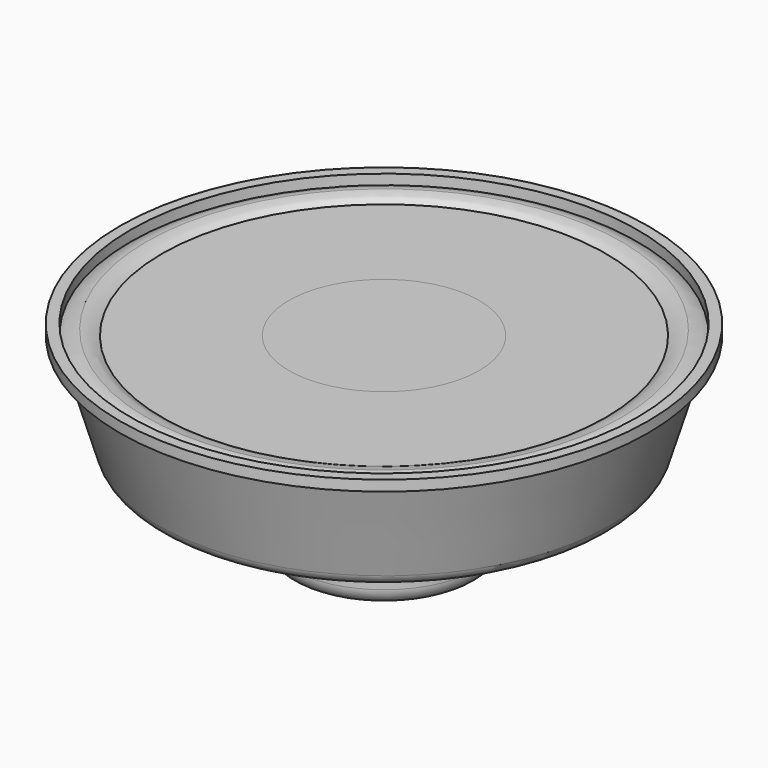
from build123d import *

# Parameters (mm, degrees)
F0_R     = 25
F0_R_2   = 24
F1_DEPTH = 1
F0_R_3   = 9
F2_DEPTH = 18
F0_R_4   = 21
F3_DEPTH = 10
F4_DEPTH = 0.5
F5_SIZE2 = 2.99999
F5_SIZE  = 9.99999
F6_R     = 1.5
F6_2_R   = 1.5


# Not quite as in the source:
# - a fillet or chamfer that OpenCascade refuses, or shapes differently, is made with other operations: its cross-section is extruded or revolved along the edge and cut away or added
# - a fillet or chamfer is up to 0.001 mm smaller than in the source, because OpenCascade refuses the exact size


with BuildPart() as f1:
    # F0 (on Top) → F1 (new body)
    with BuildSketch(Plane.XY):
        Circle(F0_R)
        Circle(F0_R_2, mode=Mode.SUBTRACT)
    extrude(amount=F1_DEPTH)

    # F0 (on Top) → F3 (join)
    with BuildSketch(Plane.XY):
        Circle(F0_R_2)
        Circle(F0_R_4, mode=Mode.SUBTRACT)
        Circle(F0_R_4)
        Circle(F0_R_3, mode=Mode.SUBTRACT)
    extrude(amount=-F3_DEPTH)

    # F5 (size 10 and 3 in the source; OpenCascade refuses exactly that, so slightly less here)
    f5_edges = [f1.edges().sort_by_distance(p)[0] for p in [
        (-24, 0, -10),
    ]]
    f5_side = f1.faces().sort_by_distance((-24, 0, -5))[0]
    chamfer(f5_edges, length=F5_SIZE, length2=F5_SIZE2, reference=f5_side)

    # F6#2
    f6_2_edges = [f1.edges().sort_by_distance(p)[0] for p in [
        (-21.00001, 0, -10),
    ]]
    fillet(f6_2_edges, radius=F6_2_R)


with BuildPart() as f2:
    # F0 (on Top) → F2 (new body)
    with BuildSketch(Plane.XY):
        Circle(F0_R_3)
    extrude(amount=-F2_DEPTH)

    # F6
    f6_edges = [f2.edges().sort_by_distance(p)[0] for p in [
        (-9, 0, -18),
    ]]
    fillet(f6_edges, radius=F6_R)


with BuildPart() as f4:
    # F0 (on Top) → F4 (new body)
    with BuildSketch(Plane.XY):
        Circle(F0_R_2)
        Circle(F0_R_4, mode=Mode.SUBTRACT)
    extrude(amount=F4_DEPTH)

    # F7: fillet of radius 2.5 on 2 edges, made by hand

    # F7_s1 → F7_t2 (revolve, cut)
    with BuildSketch(Plane.XZ):
        with BuildLine():
            ThreePointArc((24, 0), (23.290569415, 0.3717082451), (22.5, 0.5))
            Line((22.5, 0.5), (22.5, 0.55))
            Line((22.5, 0.55), (24, 0.55))
            Line((24, 0.55), (24.05, 0.5))
            ThreePointArc((24.05, 0.5), (24.05, 0.25), (24.03, 0.04))
            Line((24.03, 0.04), (24, 0))
        make_face()
    revolve(axis=Axis((0, 0, 0.5), (0, 0, 1)), mode=Mode.SUBTRACT)

    # F7_s3 → F7_t4 (revolve, cut)
    with BuildSketch(Plane.XZ):
        with BuildLine():
            ThreePointArc((21, 0), (21.709430585, 0.3717082451), (22.5, 0.5))
            Line((22.5, 0.5), (22.5, 0.55))
            Line((22.5, 0.55), (21, 0.55))
            Line((21, 0.55), (20.95, 0.5))
            ThreePointArc((20.95, 0.5), (20.95, 0.25), (20.97, 0.04))
            Line((20.97, 0.04), (21, 0))
        make_face()
    revolve(axis=Axis((0, 0, 0.5), (0, 0, 1)), mode=Mode.SUBTRACT)


solid = Compound([f1.part, f2.part, f4.part])
